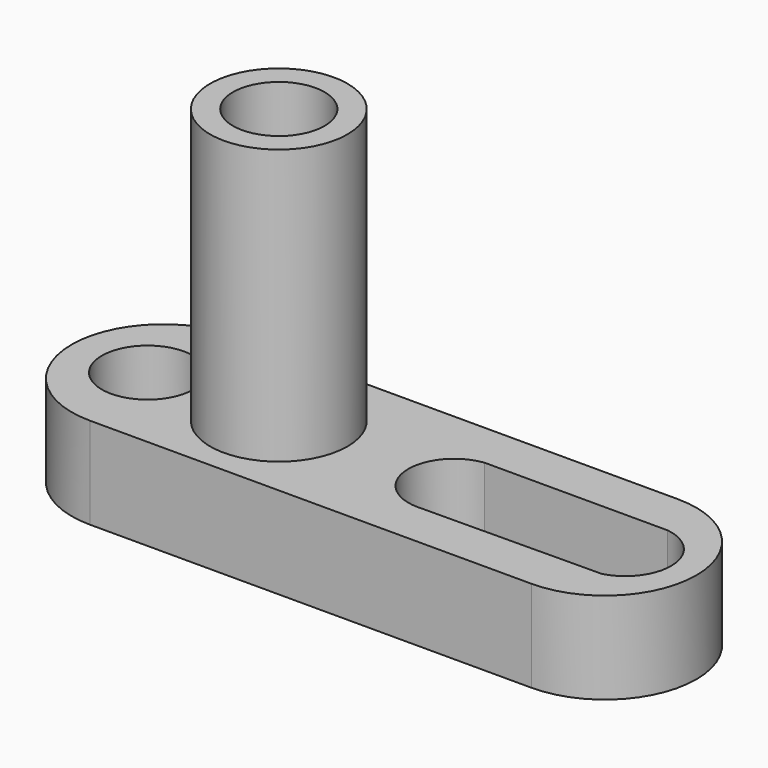
from build123d import *

# Parameters (mm, degrees)
F0_W      = 101.6
F0_H      = 12.7
F1_DEPTH  = 25.4
F2_R      = 6.35
F3_DEPTH  = 25.4
F4_R      = 9.525
F5_DEPTH  = 38.1
F6_R      = 6.35
F7_DEPTH  = 50.8
F9_DEPTH  = 25.4
F11_DEPTH = 25.4
F13_DEPTH = 25.4


with BuildPart() as f1:
    # F0 (on Front) → F1 (new body)
    with BuildSketch(Plane.XZ):
        with Locations((50.8, 6.35)):
            Rectangle(F0_W, F0_H)
    extrude(amount=F1_DEPTH)

    # F2 (on face) → F3 (cut)
    with BuildSketch(Plane.XY.offset(12.7)):
        with Locations((12.7, -12.7)):
            Circle(F2_R)
    extrude(amount=-F3_DEPTH, mode=Mode.SUBTRACT)

    # F4 (on face) → F5 (join)
    with BuildSketch(Plane.XY.offset(12.7)):
        with Locations((30.8962874115, -12.7)):
            Circle(F4_R)
    extrude(amount=F5_DEPTH)

    # F6 (on face) → F7 (cut)
    with BuildSketch(Plane.XY.offset(50.8)):
        with Locations((30.8962874115, -12.7)):
            Circle(F6_R)
    extrude(amount=-F7_DEPTH, mode=Mode.SUBTRACT)

    # F8 (on face) → F9 (cut)
    with BuildSketch(Plane.XY.offset(12.7)):
        with BuildLine():
            ThreePointArc((61.5597656887, -12.7), (59.6998937492, -17.1901280605), (55.2097656887, -19.05))
            Line((55.2097656887, -19.05), (77.399272464, -18.8575478586))
            ThreePointArc((77.399272464, -18.8575478586), (72.6114019876, -12.3324709451), (78.1212527055, -6.4044124523))
            Line((78.1212527055, -6.4044124523), (56.0392700164, -6.4044124523))
            ThreePointArc((56.0392700164, -6.4044124523), (59.9841689227, -8.5134054699), (61.5597656887, -12.7))
        make_face()
        with BuildLine():
            Line((56.0392700164, -6.4044124523), (54.3802613609, -6.4044124523))
            ThreePointArc((54.3802613609, -6.4044124523), (48.8733834035, -13.1156435206), (55.2097656887, -19.05))
            ThreePointArc((55.2097656887, -19.05), (59.6998937492, -17.1901280605), (61.5597656887, -12.7))
            ThreePointArc((61.5597656887, -12.7), (59.9841689227, -8.5134054699), (56.0392700164, -6.4044124523))
        make_face()
        with BuildLine():
            ThreePointArc((78.1212527055, -6.4044124523), (72.6114019876, -12.3324709451), (77.399272464, -18.8575478586))
            Line((77.399272464, -18.8575478586), (80.6088104115, -18.8297111673))
            ThreePointArc((80.6088104115, -18.8297111673), (83.9931343967, -16.5596541975), (85.3007570332, -12.7))
            ThreePointArc((85.3007570332, -12.7), (83.7251602672, -8.5134054699), (79.7802613609, -6.4044124523))
            Line((79.7802613609, -6.4044124523), (78.1212527055, -6.4044124523))
        make_face()
    extrude(amount=-F9_DEPTH, mode=Mode.SUBTRACT)

    # F10 (on face) → F11 (cut)
    with BuildSketch(Plane.XY.offset(12.7)):
        with BuildLine():
            ThreePointArc((76.106920933, 0), (88.806920933, -12.7), (76.106920933, -25.4))
            Line((76.106920933, -25.4), (101.6, -25.4))
            Line((101.6, -25.4), (101.6, 0))
            Line((101.6, 0), (76.106920933, 0))
        make_face()
    extrude(amount=-F11_DEPTH, mode=Mode.SUBTRACT)

    # F12 (on face) → F13 (cut)
    with BuildSketch(Plane.XY.offset(12.7)):
        with BuildLine():
            ThreePointArc((14.8660039439, -25.4), (2.1660039439, -12.7), (14.8660039439, 0))
            Line((14.8660039439, 0), (0, 0))
            Line((0, 0), (0, -25.4))
            Line((0, -25.4), (14.8660039439, -25.4))
        make_face()
    extrude(amount=-F13_DEPTH, mode=Mode.SUBTRACT)


solid = f1.part
